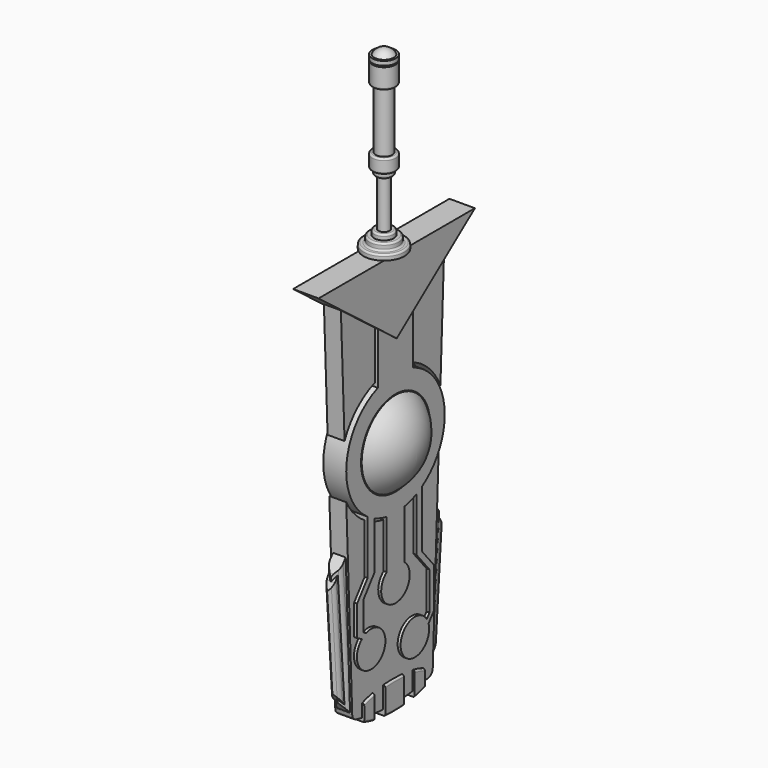
from build123d import *

# Parameters (mm, degrees)
F1_DEPTH       = 3.81
F6_DEPTH       = 2.54
F8_DEPTH       = 1.905
F10_DEPTH      = 1.27
F12_DEPTH      = 3.175
F14_R          = 19.4292744408
F14_R_2        = 18.415
F15_DEPTH      = 5.08
F19_DEPTH      = 3.429
F24_R          = 12.8743329009
F24_R_2        = 12.6424620479
F25_DEPTH      = 1.27
F28_R          = 0.508
F29_T1_DEPTH   = 35.5126267964
F29_T3_DEPTH   = 35.5126267964
F29_T8_DEPTH   = 43.5778406239
F29_T14_DEPTH  = 43.5778406239
F29_T20_DEPTH  = 43.5778406239
F29_T27_DEPTH  = 43.5778406239
F29_T33_DEPTH  = 43.5778406239
F29_T39_DEPTH  = 43.5778406239
F29_T45_DEPTH  = 43.5778406239
F29_T51_DEPTH  = 43.5778406239
F29_T58_DEPTH  = 43.5778406239
F29_T64_DEPTH  = 43.5778406239
F29_T70_DEPTH  = 43.5778406239
F29_T76_DEPTH  = 43.5778406239
F29_T82_DEPTH  = 43.5778406239
F29_T89_DEPTH  = 43.5778406239
F29_T95_DEPTH  = 43.5778406239
F29_T101_DEPTH = 43.5778406239
F29_T107_DEPTH = 43.5778406239
F29_T113_DEPTH = 43.5778406239
F29_T120_DEPTH = 43.5778406239
F29_T126_DEPTH = 43.5778406239
F30_R          = 0.508
F31_R          = 1.778


# Not quite as in the source:
# - a fillet or chamfer that OpenCascade refuses, or shapes differently, is made with other operations: its cross-section is extruded or revolved along the edge and cut away or added
# - a feature names something its author has since deleted; it is built from what else it names


with BuildPart() as f1:
    # F0 (on Right) → F1 (new body, symmetric)
    with BuildSketch(Plane.YZ):
        Polygon((0, 61.229582876), (-29.2335897684, 61.229582876), (0, 38.8180017471), (29.2335897684, 61.229582876), align=None)
    extrude(amount=F1_DEPTH, both=True)

    # F3 (on Right) → F4 (revolve)
    with BuildSketch(Plane.YZ):
        with BuildLine():
            Line((-6.1364490539, 61.229582876), (0, 61.229582876))
            Line((0, 61.229582876), (0, 114.1549376053))
            ThreePointArc((0, 114.1549376053), (-1.677015219, 113.699444169), (-2.8931638226, 112.458139658))
            Line((-2.8931638226, 112.458139658), (-3.5008313134, 112.458139658))
            Line((-3.5008313134, 112.458139658), (-3.5008313134, 111.2130246248))
            Line((-3.5008313134, 111.2130246248), (-2.9749742604, 111.2130246248))
            Line((-2.9749742604, 111.2130246248), (-2.9749742604, 110.7980277486))
            Line((-2.9749742604, 110.7980277486), (-3.5008313134, 110.7980277486))
            Line((-3.5008313134, 110.7980277486), (-3.5008313134, 104.7310199685))
            Line((-3.5008313134, 104.7310199685), (-2.4548028596, 104.7310199685))
            Line((-2.4548028596, 104.7310199685), (-2.4548028596, 86.7087509579))
            Line((-2.4548028596, 86.7087509579), (-3.5008313134, 86.7087509579))
            Line((-3.5008313134, 86.7087509579), (-3.5008313134, 82.5219493456))
            Line((-3.5008313134, 82.5219493456), (-2.5814441033, 82.5219493456))
            Line((-2.5814441033, 82.5219493456), (-2.5814441033, 80.8570649571))
            Line((-2.5814441033, 80.8570649571), (-1.6710797196, 80.8570649571))
            Line((-1.6710797196, 80.8570649571), (-1.6710797196, 66.452437882))
            Line((-1.6710797196, 66.452437882), (-2.9182097047, 66.452437882))
            Line((-2.9182097047, 66.452437882), (-2.9182097047, 64.8802369833))
            Line((-2.9182097047, 64.8802369833), (-4.3904725462, 64.8802369833))
            Line((-4.3904725462, 64.8802369833), (-4.3904725462, 62.8347471356))
            Line((-4.3904725462, 62.8347471356), (-6.1364490539, 62.8347471356))
            Line((-6.1364490539, 62.8347471356), (-6.1364490539, 61.229582876))
        make_face()
    revolve(axis=Axis((0, 0, -49.0248562196), (0, 0, 1)))

    # F5 (on Right) → F6 (join, symmetric)
    with BuildSketch(Plane.YZ):
        with BuildLine():
            Line((0, 38.8180017471), (-19.2966815204, 53.6115712963))
            Line((-19.2966815204, 53.6115712963), (-14.9982394651, -56.0456514359))
            ThreePointArc((-14.9982394651, -56.0456514359), (0, -58.042105807), (14.9982394651, -56.0456514359))
            Line((14.9982394651, -56.0456514359), (19.2966815204, 53.6115712963))
            Line((19.2966815204, 53.6115712963), (0, 38.8180017471))
        make_face()
    extrude(amount=F6_DEPTH, both=True)

    # F7 (on Right) → F8 (join, symmetric)
    with BuildSketch(Plane.YZ):
        Polygon((-15.0661740028, -54.3125786982), (-16.6965185978, -12.7209838658), (-20.0156738163, -16.8685576027), (-17.5727236001, -51.2147228941), align=None)
        Polygon((20.0156738163, -16.8685576027), (16.6965185978, -12.7209838658), (15.0661740028, -54.3125786982), (17.5727236001, -51.2147228941), align=None)
    extrude(amount=F8_DEPTH, both=True)

    # F9 (on Right) → F10 (join, symmetric)
    with BuildSketch(Plane.YZ):
        Polygon((-17.6375055068, -50.3039347575), (-19.9093083474, -18.3639814359), (-21.7317498197, -21.2546187948), (-19.8610109278, -47.5558945106), align=None)
        Polygon((21.7317498197, -21.2546187948), (19.9093083474, -18.3639814359), (17.6375055068, -50.3039347575), (19.8610109278, -47.5558945106), align=None)
    extrude(amount=F10_DEPTH, both=True)

    # F11 (on Right) → F12 (join, symmetric)
    with BuildSketch(Plane.YZ):
        with BuildLine():
            Line((-11.3537593797, -53.0362920111), (-11.3537593797, -57.9446920642))
            add(Edge.make_bspline(
                [(-11.3537593797, -57.9446920642), (-9.7769390699, -58.5898523746), (-7.511371281, -59.016674757)],
                knots=[3.7701097937, 3.7701097937, 3.7701097937, 4.1477051693, 4.1477051693, 4.1477051693], degree=2, weights=[1, 0.9822305926, 1]))
            Line((-7.511371281, -59.016674757), (-7.511371281, -51.9643093183))
            add(Edge.make_bspline(
                [(-7.511371281, -51.9643093183), (-9.7769390699, -52.3911317007), (-11.3537593797, -53.0362920111)],
                knots=[2.1354801378, 2.1354801378, 2.1354801378, 2.5130755135, 2.5130755135, 2.5130755135], degree=2, weights=[1, 0.9822305926, 1]))
        make_face()
        with BuildLine():
            add(Edge.make_bspline(
                [(0, -51.31629855), (-1.775820711, -51.31629855), (-3.4956861232, -51.4478254786)],
                knots=[1.5707963268, 1.5707963268, 1.5707963268, 1.8224962383, 1.8224962383, 1.8224962383], degree=2, weights=[1, 0.9920913408, 1]))
            Line((-3.4956861232, -51.4478254786), (-3.4956861232, -59.5331585967))
            add(Edge.make_bspline(
                [(-3.4956861232, -59.5331585967), (-1.775820711, -59.6646855253), (0, -59.6646855253)],
                knots=[4.4606890689, 4.4606890689, 4.4606890689, 4.7123889804, 4.7123889804, 4.7123889804], degree=2, weights=[1, 0.9920913408, 1]))
            Line((0, -59.6646855253), (0, -51.31629855))
        make_face()
        with BuildLine():
            add(Edge.make_bspline(
                [(3.4956861232, -51.4478254786), (1.775820711, -51.31629855), (0, -51.31629855)],
                knots=[4.4606890689, 4.4606890689, 4.4606890689, 4.7123889804, 4.7123889804, 4.7123889804], degree=2, weights=[1, 0.9920913408, 1]))
            Line((0, -51.31629855), (0, -59.6646855253))
            add(Edge.make_bspline(
                [(0, -59.6646855253), (1.775820711, -59.6646855253), (3.4956861232, -59.5331585967)],
                knots=[1.5707963268, 1.5707963268, 1.5707963268, 1.8224962383, 1.8224962383, 1.8224962383], degree=2, weights=[1, 0.9920913408, 1]))
            Line((3.4956861232, -59.5331585967), (3.4956861232, -51.4478254786))
        make_face()
        with BuildLine():
            add(Edge.make_bspline(
                [(11.3537593797, -53.0362920111), (9.7769390699, -52.3911317007), (7.511371281, -51.9643093183)],
                knots=[3.7701097937, 3.7701097937, 3.7701097937, 4.1477051693, 4.1477051693, 4.1477051693], degree=2, weights=[1, 0.9822305926, 1]))
            Line((7.511371281, -51.9643093183), (7.511371281, -59.016674757))
            add(Edge.make_bspline(
                [(7.511371281, -59.016674757), (9.7769390699, -58.5898523746), (11.3537593797, -57.9446920642)],
                knots=[2.1354801378, 2.1354801378, 2.1354801378, 2.5130755135, 2.5130755135, 2.5130755135], degree=2, weights=[1, 0.9822305926, 1]))
            Line((11.3537593797, -57.9446920642), (11.3537593797, -53.0362920111))
        make_face()
    extrude(amount=F12_DEPTH, both=True)

    # F14 (on face) → F15 (cut, through all)
    with BuildSketch(Plane(origin=(-2.54, 0, 0), x_dir=(0, -1, 0), z_dir=(-1, 0, 0))):
        with Locations((0, 11.139294037)):
            Circle(F14_R)
        with Locations((0, 11.139294037)):
            Circle(F14_R_2, mode=Mode.SUBTRACT)
    extrude(amount=-F15_DEPTH, mode=Mode.SUBTRACT)

    # F18 (on Right) + F17 (on Right) + F16 (on Right) + F13 (on Right) → F19 (join, symmetric)
    with BuildSketch(Plane.YZ):
        with BuildLine():
            Line((9.9362479523, -21.4804578573), (9.9362479523, -4.3650021944))
            ThreePointArc((9.9362479523, -4.3650021944), (8.9028503726, -4.9806153996), (7.831467, -5.527449785))
            Line((7.831467, -5.527449785), (7.831467, -21.4804578573))
            Line((7.831467, -21.4804578573), (12.7164591104, -27.3665288538))
            Line((12.7164591104, -27.3665288538), (12.7164591104, -38.7271232903))
            Line((12.7164591104, -38.7271232903), (11.709224863, -39.9957729418))
            ThreePointArc((11.709224863, -39.9957729418), (12.0953554466, -40.6866533588), (12.3750045896, -41.427064687))
            Line((12.3750045896, -41.427064687), (14.3657037988, -38.9197036985))
            Line((14.3657037988, -38.9197036985), (14.3657037988, -26.8176397809))
            Line((14.3657037988, -26.8176397809), (9.9362479523, -21.4804578573))
        make_face()
        with BuildLine():
            ThreePointArc((12.5929859714, -42.936339181), (12.5382093664, -42.1738719062), (12.3750045896, -41.427064687))
            ThreePointArc((12.3750045896, -41.427064687), (12.0953554466, -40.6866533588), (11.709224863, -39.9957729418))
            ThreePointArc((11.709224863, -39.9957729418), (2.1507020008, -44.4715886318), (12.5929859714, -42.936339181))
        make_face()
    with BuildSketch(Plane.YZ):
        with BuildLine():
            Line((-7.831467, -19.77381139), (-7.831467, -5.527449785))
            ThreePointArc((-7.831467, -5.527449785), (-9.1665508867, -4.8321357625), (-10.4403848891, -4.0301024035))
            Line((-10.4403848891, -4.0301024035), (-10.4403848891, -20.2001390615))
            Line((-10.4403848891, -20.2001390615), (-14.3241826304, -25.3432573233))
            Line((-14.3241826304, -25.3432573233), (-14.3241826304, -34.4560037236))
            Line((-14.3241826304, -34.4560037236), (-12.5747991422, -35.4090025638))
            ThreePointArc((-12.5747991422, -35.4090025638), (-11.8159129933, -34.8635845591), (-10.9734812348, -34.4589888114))
            Line((-10.9734812348, -34.4589888114), (-11.9662850956, -33.9181463178))
            Line((-11.9662850956, -33.9181463178), (-11.9662850956, -25.249343298))
            Line((-11.9662850956, -25.249343298), (-7.831467, -19.77381139))
        make_face()
        with BuildLine():
            ThreePointArc((-3.7603277346, -39.4510162675), (-6.0588581474, -35.0649610484), (-10.9734812348, -34.4589888114))
            ThreePointArc((-10.9734812348, -34.4589888114), (-11.8159129933, -34.8635845591), (-12.5747991422, -35.4090025638))
            ThreePointArc((-12.5747991422, -35.4090025638), (-11.3176947209, -44.2995413261), (-3.7603277346, -39.4510162675))
        make_face()
    with BuildSketch(Plane.YZ):
        with BuildLine():
            Line((3.3077583424, -21.54598683), (3.3077583424, -6.9761954609))
            ThreePointArc((3.3077583424, -6.9761954609), (0, -7.275705963), (-3.3077583424, -6.9761954609))
            Line((-3.3077583424, -6.9761954609), (-3.3077583424, -21.54598683))
            ThreePointArc((-3.3077583424, -21.54598683), (0, -20.3965167615), (3.3077583424, -21.54598683))
        make_face()
        with BuildLine():
            ThreePointArc((5.334, -25.7305167615), (4.8007884247, -23.4058691537), (3.3077583424, -21.54598683))
            ThreePointArc((3.3077583424, -21.54598683), (0, -20.3965167615), (-3.3077583424, -21.54598683))
            ThreePointArc((-3.3077583424, -21.54598683), (-2.3246476079, -30.5313051863), (5.334, -25.7305167615))
        make_face()
    with BuildSketch(Plane.YZ):
        with BuildLine():
            ThreePointArc((-6.5928324384, 28.3336764172), (-10.433245316, -4.035013762), (18.415, 11.139294037))
            ThreePointArc((18.415, 11.139294037), (15.1743077989, 21.5725393529), (6.5928324384, 28.3336764172))
            ThreePointArc((6.5928324384, 28.3336764172), (0, 29.554294037), (-6.5928324384, 28.3336764172))
        make_face()
        with BuildLine():
            ThreePointArc((-6.5928324384, 28.3336764172), (0, 29.554294037), (6.5928324384, 28.3336764172))
            Line((6.5928324384, 28.3336764172), (6.5928324384, 43.8723176978))
            Line((6.5928324384, 43.8723176978), (0, 38.8180017471))
            Line((0, 38.8180017471), (-6.5928324384, 43.8723176978))
            Line((-6.5928324384, 43.8723176978), (-6.5928324384, 28.3336764172))
        make_face()
    extrude(amount=F19_DEPTH, both=True)

    # F21 (on Front) → F22 (revolve)
    with BuildSketch(Plane.XZ):
        with BuildLine():
            Line((3.429, 11.139294037), (3.429, -1.5031680109))
            ThreePointArc((3.429, -1.5031680109), (8.1433373008, 4.0524935149), (9.8367390651, 11.139294037))
            Line((9.8367390651, 11.139294037), (3.429, 11.139294037))
        make_face()
    revolve(axis=Axis((6.6328695326, 0, 11.139294037), (1, 0, 0)))

    # F23: F1 across plane


with BuildPart() as f1_1:
    add(f1.part)
    add(f1.part.mirror(Plane.YZ))

    # F26: F25 across plane


with BuildPart() as f25:
    # F24 (on face) → F25 (new body)
    with BuildSketch(Plane(origin=(-3.429, 0, 0), x_dir=(0, -1, 0), z_dir=(-1, 0, 0))):
        with Locations((0, 11.139294037)):
            Circle(F24_R)
        with Locations((0, 11.139294037)):
            Circle(F24_R_2, mode=Mode.SUBTRACT)
    extrude(amount=-F25_DEPTH)


with BuildPart() as f1_2:
    add(f1_1.part)
    add(f25.part.mirror(Plane.YZ), mode=Mode.SUBTRACT)

    # F27: cut F25
    add(f25.part, mode=Mode.SUBTRACT)

    # F28
    f28_edges = [f1_2.edges().sort_by_distance(p)[0] for p in [
        (3.175, 0, -59.664686),
        (3.175, 9.459102, -58.574423),
        (3.175, -9.459102, -58.574423),
        (-3.175, 9.459102, -58.574423),
        (-3.175, 0, -59.664686),
        (-3.175, -9.459102, -58.574423),
        (3.175, -9.459102, -52.406561),
        (3.175, 0, -51.316299),
        (3.175, 9.459102, -52.406561),
        (-3.175, -9.459102, -52.406561),
        (-3.175, 0, -51.316299),
        (-3.175, 9.459102, -52.406561),
    ]]
    fillet(f28_edges, radius=F28_R)

    # F29: chamfer of 1.778 on 8 edges, made by hand

    # F29_s2 → F29_t1 (cut)
    with BuildSketch(Plane(origin=(0, 1.0703778238, -15.0487608862), x_dir=(1, 0, 0), z_dir=(0, 0.0709480662, -0.9974800108))):
        Polygon((-1.27, 21.4069601452), (0.508, 23.1849601452), (-1.27, 23.1849601452), align=None)
        Polygon((1.27, 21.4069601452), (-0.508, 23.1849601452), (1.27, 23.1849601452), align=None)
    extrude(amount=F29_T1_DEPTH, mode=Mode.SUBTRACT)

    # F29_s4 → F29_t3 (cut)
    with BuildSketch(Plane(origin=(0, -3.5899300198, -50.4718962459), x_dir=(1, 0, 0), z_dir=(0, 0.0709480662, 0.9974800108))):
        Polygon((-1.27, 21.4069601452), (0.508, 23.1849601452), (-1.27, 23.1849601452), align=None)
        Polygon((1.27, 21.4069601452), (-0.508, 23.1849601452), (1.27, 23.1849601452), align=None)
    extrude(amount=F29_T3_DEPTH, mode=Mode.SUBTRACT)


with BuildPart() as f29_tool6:
    # F29_s7 → F29_t8 (new body)
    with BuildSketch(Plane(origin=(0, 0.7686175292, -10.8062229544), x_dir=(1, 0, 0), z_dir=(0, 0.0709480662, -0.9974800108))):
        Polygon((1.905, 19.3840260751), (0.127, 21.1620260751), (1.905, 21.1620260751), align=None)
    extrude(amount=F29_T8_DEPTH)

    split(bisect_by=Plane(origin=(0, -5.9617754982, 3.7586821063), x_dir=(1, 0, 0), z_dir=(0, -0.8459146267, 0.5333183331)), keep=Keep.TOP)

    split(bisect_by=Plane.YZ.offset(1.27), keep=Keep.TOP)


with BuildPart() as f1_3:
    add(f1_2.part)

    # F29_t5: cut F29_tool6
    add(f29_tool6.part, mode=Mode.SUBTRACT)


with BuildPart() as f29_tool12:
    # F29_s13 → F29_t14 (new body)
    with BuildSketch(Plane(origin=(0, 0.7686175292, -10.8062229544), x_dir=(1, 0, 0), z_dir=(0, 0.0709480662, -0.9974800108))):
        Polygon((1.905, 19.3840260751), (0.127, 21.1620260751), (1.905, 21.1620260751), align=None)
    extrude(amount=F29_T14_DEPTH)

    split(bisect_by=Plane(origin=(0, -5.9617754982, 3.7586821063), x_dir=(1, 0, 0), z_dir=(0, -0.8459146267, 0.5333183331)), keep=Keep.TOP)

    split(bisect_by=Plane.YZ.offset(1.27), keep=Keep.BOTTOM)


with BuildPart() as f1_4:
    add(f1_3.part)

    # F29_t11: cut F29_tool12
    add(f29_tool12.part, mode=Mode.SUBTRACT)


with BuildPart() as f29_tool18:
    # F29_s19 → F29_t20 (new body)
    with BuildSketch(Plane(origin=(0, 0.7686175292, -10.8062229544), x_dir=(1, 0, 0), z_dir=(0, 0.0709480662, -0.9974800108))):
        Polygon((1.905, 19.3840260751), (0.127, 21.1620260751), (1.905, 21.1620260751), align=None)
    extrude(amount=F29_T20_DEPTH)

    split(bisect_by=Plane(origin=(0, -5.9617754982, 3.7586821063), x_dir=(1, 0, 0), z_dir=(0, 0.8459146267, -0.5333183331)), keep=Keep.TOP)

    split(bisect_by=Plane(origin=(0, -35.2573114289, -28.5275381909), x_dir=(1, 0, 0), z_dir=(0, 0.7773968328, 0.6290104644)), keep=Keep.TOP)

    split(bisect_by=Plane.YZ.offset(1.27), keep=Keep.TOP)


with BuildPart() as f1_5:
    add(f1_4.part)

    # F29_t17: cut F29_tool18
    add(f29_tool18.part, mode=Mode.SUBTRACT)


with BuildPart() as f29_tool25:
    # F29_s26 → F29_t27 (new body)
    with BuildSketch(Plane(origin=(0, 0.7686175292, -10.8062229544), x_dir=(1, 0, 0), z_dir=(0, 0.0709480662, -0.9974800108))):
        Polygon((1.905, 19.3840260751), (0.127, 21.1620260751), (1.905, 21.1620260751), align=None)
    extrude(amount=F29_T27_DEPTH)

    split(bisect_by=Plane(origin=(0, -35.2573114289, -28.5275381909), x_dir=(1, 0, 0), z_dir=(0, -0.7773968328, -0.6290104644)), keep=Keep.TOP)

    split(bisect_by=Plane.YZ.offset(1.27), keep=Keep.TOP)


with BuildPart() as f1_6:
    add(f1_5.part)

    # F29_t24: cut F29_tool25
    add(f29_tool25.part, mode=Mode.SUBTRACT)


with BuildPart() as f29_tool31:
    # F29_s32 → F29_t33 (new body)
    with BuildSketch(Plane(origin=(0, 0.7686175292, -10.8062229544), x_dir=(1, 0, 0), z_dir=(0, 0.0709480662, -0.9974800108))):
        Polygon((1.905, 19.3840260751), (0.127, 21.1620260751), (1.905, 21.1620260751), align=None)
    extrude(amount=F29_T33_DEPTH)

    split(bisect_by=Plane(origin=(0, -35.2573114289, -28.5275381909), x_dir=(1, 0, 0), z_dir=(0, -0.7773968328, -0.6290104644)), keep=Keep.TOP)

    split(bisect_by=Plane.YZ.offset(1.27), keep=Keep.BOTTOM)


with BuildPart() as f1_7:
    add(f1_6.part)

    # F29_t30: cut F29_tool31
    add(f29_tool31.part, mode=Mode.SUBTRACT)


with BuildPart() as f29_tool37:
    # F29_s38 → F29_t39 (new body)
    with BuildSketch(Plane(origin=(0, 0.7686175292, -10.8062229544), x_dir=(1, 0, 0), z_dir=(0, 0.0709480662, -0.9974800108))):
        Polygon((-1.905, 19.3840260751), (-0.127, 21.1620260751), (-1.905, 21.1620260751), align=None)
    extrude(amount=F29_T39_DEPTH)

    split(bisect_by=Plane(origin=(0, -5.9617754982, 3.7586821063), x_dir=(1, 0, 0), z_dir=(0, -0.8459146267, 0.5333183331)), keep=Keep.TOP)

    split(bisect_by=Plane.YZ.offset(-1.27), keep=Keep.BOTTOM)


with BuildPart() as f1_8:
    add(f1_7.part)

    # F29_t36: cut F29_tool37
    add(f29_tool37.part, mode=Mode.SUBTRACT)


with BuildPart() as f29_tool43:
    # F29_s44 → F29_t45 (new body)
    with BuildSketch(Plane(origin=(0, 0.7686175292, -10.8062229544), x_dir=(1, 0, 0), z_dir=(0, 0.0709480662, -0.9974800108))):
        Polygon((-1.905, 19.3840260751), (-0.127, 21.1620260751), (-1.905, 21.1620260751), align=None)
    extrude(amount=F29_T45_DEPTH)

    split(bisect_by=Plane(origin=(0, -5.9617754982, 3.7586821063), x_dir=(1, 0, 0), z_dir=(0, -0.8459146267, 0.5333183331)), keep=Keep.TOP)

    split(bisect_by=Plane.YZ.offset(-1.27), keep=Keep.TOP)


with BuildPart() as f1_9:
    add(f1_8.part)

    # F29_t42: cut F29_tool43
    add(f29_tool43.part, mode=Mode.SUBTRACT)


with BuildPart() as f29_tool49:
    # F29_s50 → F29_t51 (new body)
    with BuildSketch(Plane(origin=(0, 0.7686175292, -10.8062229544), x_dir=(1, 0, 0), z_dir=(0, 0.0709480662, -0.9974800108))):
        Polygon((-1.905, 19.3840260751), (-0.127, 21.1620260751), (-1.905, 21.1620260751), align=None)
    extrude(amount=F29_T51_DEPTH)

    split(bisect_by=Plane(origin=(0, -5.9617754982, 3.7586821063), x_dir=(1, 0, 0), z_dir=(0, 0.8459146267, -0.5333183331)), keep=Keep.TOP)

    split(bisect_by=Plane.YZ.offset(-1.27), keep=Keep.BOTTOM)

    split(bisect_by=Plane(origin=(0, -35.2573114289, -28.5275381909), x_dir=(1, 0, 0), z_dir=(0, 0.7773968328, 0.6290104644)), keep=Keep.TOP)


with BuildPart() as f1_10:
    add(f1_9.part)

    # F29_t48: cut F29_tool49
    add(f29_tool49.part, mode=Mode.SUBTRACT)


with BuildPart() as f29_tool56:
    # F29_s57 → F29_t58 (new body)
    with BuildSketch(Plane(origin=(0, 0.7686175292, -10.8062229544), x_dir=(1, 0, 0), z_dir=(0, 0.0709480662, -0.9974800108))):
        Polygon((-1.905, 19.3840260751), (-0.127, 21.1620260751), (-1.905, 21.1620260751), align=None)
    extrude(amount=F29_T58_DEPTH)

    split(bisect_by=Plane.YZ.offset(-1.27), keep=Keep.BOTTOM)

    split(bisect_by=Plane(origin=(0, -35.2573114289, -28.5275381909), x_dir=(1, 0, 0), z_dir=(0, -0.7773968328, -0.6290104644)), keep=Keep.TOP)


with BuildPart() as f1_11:
    add(f1_10.part)

    # F29_t55: cut F29_tool56
    add(f29_tool56.part, mode=Mode.SUBTRACT)


with BuildPart() as f29_tool62:
    # F29_s63 → F29_t64 (new body)
    with BuildSketch(Plane(origin=(0, 0.7686175292, -10.8062229544), x_dir=(1, 0, 0), z_dir=(0, 0.0709480662, -0.9974800108))):
        Polygon((-1.905, 19.3840260751), (-0.127, 21.1620260751), (-1.905, 21.1620260751), align=None)
    extrude(amount=F29_T64_DEPTH)

    split(bisect_by=Plane.YZ.offset(-1.27), keep=Keep.TOP)

    split(bisect_by=Plane(origin=(0, -35.2573114289, -28.5275381909), x_dir=(1, 0, 0), z_dir=(0, -0.7773968328, -0.6290104644)), keep=Keep.TOP)


with BuildPart() as f1_12:
    add(f1_11.part)

    # F29_t61: cut F29_tool62
    add(f29_tool62.part, mode=Mode.SUBTRACT)


with BuildPart() as f29_tool68:
    # F29_s69 → F29_t70 (new body)
    with BuildSketch(Plane(origin=(0, -3.8603810495, -54.2742478897), x_dir=(1, 0, 0), z_dir=(0, 0.0709480662, 0.9974800108))):
        Polygon((-1.905, 19.3840260751), (-0.127, 21.1620260751), (-1.905, 21.1620260751), align=None)
    extrude(amount=F29_T70_DEPTH)

    split(bisect_by=Plane(origin=(0, 35.2573114289, -28.5275381909), x_dir=(1, 0, 0), z_dir=(0, 0.7773968328, -0.6290104644)), keep=Keep.TOP)

    split(bisect_by=Plane.YZ.offset(-1.27), keep=Keep.BOTTOM)


with BuildPart() as f1_13:
    add(f1_12.part)

    # F29_t67: cut F29_tool68
    add(f29_tool68.part, mode=Mode.SUBTRACT)


with BuildPart() as f29_tool74:
    # F29_s75 → F29_t76 (new body)
    with BuildSketch(Plane(origin=(0, -3.8603810495, -54.2742478897), x_dir=(1, 0, 0), z_dir=(0, 0.0709480662, 0.9974800108))):
        Polygon((-1.905, 19.3840260751), (-0.127, 21.1620260751), (-1.905, 21.1620260751), align=None)
    extrude(amount=F29_T76_DEPTH)

    split(bisect_by=Plane(origin=(0, 35.2573114289, -28.5275381909), x_dir=(1, 0, 0), z_dir=(0, 0.7773968328, -0.6290104644)), keep=Keep.TOP)

    split(bisect_by=Plane.YZ.offset(-1.27), keep=Keep.TOP)


with BuildPart() as f1_14:
    add(f1_13.part)

    # F29_t73: cut F29_tool74
    add(f29_tool74.part, mode=Mode.SUBTRACT)


with BuildPart() as f29_tool80:
    # F29_s81 → F29_t82 (new body)
    with BuildSketch(Plane(origin=(0, -3.8603810495, -54.2742478897), x_dir=(1, 0, 0), z_dir=(0, 0.0709480662, 0.9974800108))):
        Polygon((-1.905, 19.3840260751), (-0.127, 21.1620260751), (-1.905, 21.1620260751), align=None)
    extrude(amount=F29_T82_DEPTH)

    split(bisect_by=Plane(origin=(0, 35.2573114289, -28.5275381909), x_dir=(1, 0, 0), z_dir=(0, -0.7773968328, 0.6290104644)), keep=Keep.TOP)

    split(bisect_by=Plane.YZ.offset(-1.27), keep=Keep.BOTTOM)

    split(bisect_by=Plane(origin=(0, 5.9617754982, 3.7586821063), x_dir=(1, 0, 0), z_dir=(0, -0.8459146267, -0.5333183331)), keep=Keep.TOP)


with BuildPart() as f1_15:
    add(f1_14.part)

    # F29_t79: cut F29_tool80
    add(f29_tool80.part, mode=Mode.SUBTRACT)


with BuildPart() as f29_tool87:
    # F29_s88 → F29_t89 (new body)
    with BuildSketch(Plane(origin=(0, -3.8603810495, -54.2742478897), x_dir=(1, 0, 0), z_dir=(0, 0.0709480662, 0.9974800108))):
        Polygon((-1.905, 19.3840260751), (-0.127, 21.1620260751), (-1.905, 21.1620260751), align=None)
    extrude(amount=F29_T89_DEPTH)

    split(bisect_by=Plane.YZ.offset(-1.27), keep=Keep.BOTTOM)

    split(bisect_by=Plane(origin=(0, 5.9617754982, 3.7586821063), x_dir=(1, 0, 0), z_dir=(0, 0.8459146267, 0.5333183331)), keep=Keep.TOP)


with BuildPart() as f1_16:
    add(f1_15.part)

    # F29_t86: cut F29_tool87
    add(f29_tool87.part, mode=Mode.SUBTRACT)


with BuildPart() as f29_tool93:
    # F29_s94 → F29_t95 (new body)
    with BuildSketch(Plane(origin=(0, -3.8603810495, -54.2742478897), x_dir=(1, 0, 0), z_dir=(0, 0.0709480662, 0.9974800108))):
        Polygon((-1.905, 19.3840260751), (-0.127, 21.1620260751), (-1.905, 21.1620260751), align=None)
    extrude(amount=F29_T95_DEPTH)

    split(bisect_by=Plane.YZ.offset(-1.27), keep=Keep.TOP)

    split(bisect_by=Plane(origin=(0, 5.9617754982, 3.7586821063), x_dir=(1, 0, 0), z_dir=(0, 0.8459146267, 0.5333183331)), keep=Keep.TOP)


with BuildPart() as f1_17:
    add(f1_16.part)

    # F29_t92: cut F29_tool93
    add(f29_tool93.part, mode=Mode.SUBTRACT)


with BuildPart() as f29_tool99:
    # F29_s100 → F29_t101 (new body)
    with BuildSketch(Plane(origin=(0, -3.8603810495, -54.2742478897), x_dir=(1, 0, 0), z_dir=(0, 0.0709480662, 0.9974800108))):
        Polygon((1.905, 19.3840260751), (0.127, 21.1620260751), (1.905, 21.1620260751), align=None)
    extrude(amount=F29_T101_DEPTH)

    split(bisect_by=Plane(origin=(0, 35.2573114289, -28.5275381909), x_dir=(1, 0, 0), z_dir=(0, 0.7773968328, -0.6290104644)), keep=Keep.TOP)

    split(bisect_by=Plane.YZ.offset(1.27), keep=Keep.TOP)


with BuildPart() as f1_18:
    add(f1_17.part)

    # F29_t98: cut F29_tool99
    add(f29_tool99.part, mode=Mode.SUBTRACT)


with BuildPart() as f29_tool105:
    # F29_s106 → F29_t107 (new body)
    with BuildSketch(Plane(origin=(0, -3.8603810495, -54.2742478897), x_dir=(1, 0, 0), z_dir=(0, 0.0709480662, 0.9974800108))):
        Polygon((1.905, 19.3840260751), (0.127, 21.1620260751), (1.905, 21.1620260751), align=None)
    extrude(amount=F29_T107_DEPTH)

    split(bisect_by=Plane(origin=(0, 35.2573114289, -28.5275381909), x_dir=(1, 0, 0), z_dir=(0, 0.7773968328, -0.6290104644)), keep=Keep.TOP)

    split(bisect_by=Plane.YZ.offset(1.27), keep=Keep.BOTTOM)


with BuildPart() as f1_19:
    add(f1_18.part)

    # F29_t104: cut F29_tool105
    add(f29_tool105.part, mode=Mode.SUBTRACT)


with BuildPart() as f29_tool111:
    # F29_s112 → F29_t113 (new body)
    with BuildSketch(Plane(origin=(0, -3.8603810495, -54.2742478897), x_dir=(1, 0, 0), z_dir=(0, 0.0709480662, 0.9974800108))):
        Polygon((1.905, 19.3840260751), (0.127, 21.1620260751), (1.905, 21.1620260751), align=None)
    extrude(amount=F29_T113_DEPTH)

    split(bisect_by=Plane(origin=(0, 35.2573114289, -28.5275381909), x_dir=(1, 0, 0), z_dir=(0, -0.7773968328, 0.6290104644)), keep=Keep.TOP)

    split(bisect_by=Plane(origin=(0, 5.9617754982, 3.7586821063), x_dir=(1, 0, 0), z_dir=(0, -0.8459146267, -0.5333183331)), keep=Keep.TOP)

    split(bisect_by=Plane.YZ.offset(1.27), keep=Keep.TOP)


with BuildPart() as f1_20:
    add(f1_19.part)

    # F29_t110: cut F29_tool111
    add(f29_tool111.part, mode=Mode.SUBTRACT)


with BuildPart() as f29_tool118:
    # F29_s119 → F29_t120 (new body)
    with BuildSketch(Plane(origin=(0, -3.8603810495, -54.2742478897), x_dir=(1, 0, 0), z_dir=(0, 0.0709480662, 0.9974800108))):
        Polygon((1.905, 19.3840260751), (0.127, 21.1620260751), (1.905, 21.1620260751), align=None)
    extrude(amount=F29_T120_DEPTH)

    split(bisect_by=Plane(origin=(0, 5.9617754982, 3.7586821063), x_dir=(1, 0, 0), z_dir=(0, 0.8459146267, 0.5333183331)), keep=Keep.TOP)

    split(bisect_by=Plane.YZ.offset(1.27), keep=Keep.TOP)


with BuildPart() as f1_21:
    add(f1_20.part)

    # F29_t117: cut F29_tool118
    add(f29_tool118.part, mode=Mode.SUBTRACT)


with BuildPart() as f29_tool124:
    # F29_s125 → F29_t126 (new body)
    with BuildSketch(Plane(origin=(0, -3.8603810495, -54.2742478897), x_dir=(1, 0, 0), z_dir=(0, 0.0709480662, 0.9974800108))):
        Polygon((1.905, 19.3840260751), (0.127, 21.1620260751), (1.905, 21.1620260751), align=None)
    extrude(amount=F29_T126_DEPTH)

    split(bisect_by=Plane(origin=(0, 5.9617754982, 3.7586821063), x_dir=(1, 0, 0), z_dir=(0, 0.8459146267, 0.5333183331)), keep=Keep.TOP)

    split(bisect_by=Plane.YZ.offset(1.27), keep=Keep.BOTTOM)


with BuildPart() as f1_22:
    add(f1_21.part)

    # F29_t123: cut F29_tool124
    add(f29_tool124.part, mode=Mode.SUBTRACT)

    # F30
    f30_edges = [f1_22.edges().sort_by_distance(p)[0] for p in [
        (0, -4.390473, 63.857492),
        (0, 4.390473, 62.834747),
        (0, 4.390473, 64.880237),
        (0, 6.136449, 62.834747),
        (0, 2.91821, 66.452438),
        (0, 3.500831, 86.708751),
        (0, 3.500831, 82.521949),
        (0, 3.500831, 104.73102),
        (0, 2.581444, 80.857065),
    ]]
    fillet(f30_edges, radius=F30_R)

    # F31
    f31_edges = [f1_22.edges().sort_by_distance(p)[0] for p in [
        (0, -14.998239, -56.045651),
        (0, 14.998239, -56.045651),
        (0, 17.572724, -51.214723),
        (0, -20.015674, -16.868558),
        (0, 20.015674, -16.868558),
        (0, -17.572724, -51.214723),
        (-1.27, -19.018346, -34.342591),
        (1.27, -19.018346, -34.342591),
        (-1.27, 19.018346, -34.342591),
        (1.27, 19.018346, -34.342591),
        (1.905, 16.998557, -34.226511),
        (-1.905, 16.998557, -34.226511),
        (1.905, -16.998557, -34.226511),
        (-1.905, -16.998557, -34.226511),
    ]]
    fillet(f31_edges, radius=F31_R)


solid = f1_22.part
